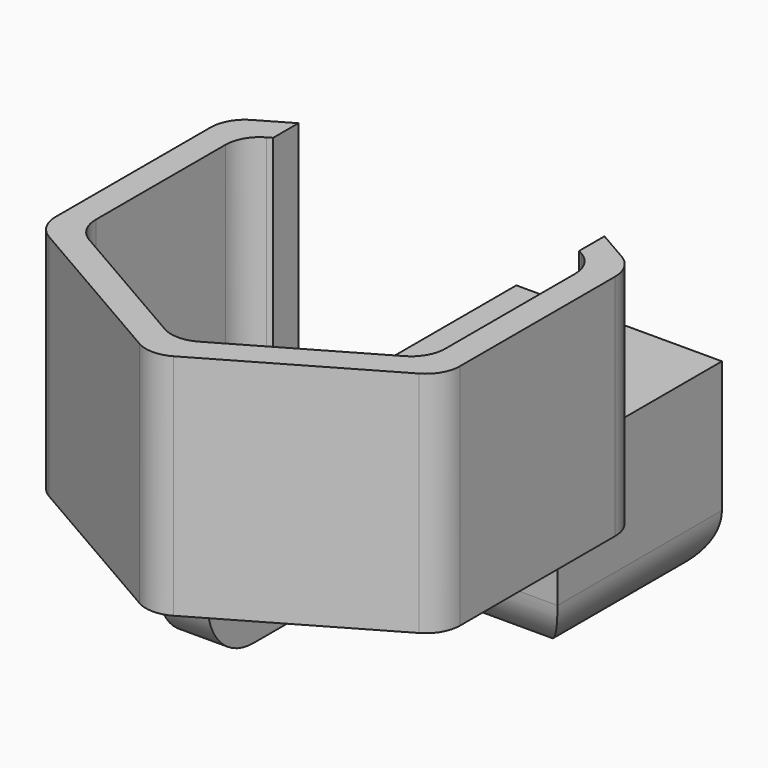
from build123d import *

# Parameters (mm, degrees)
F1_DEPTH     = 1.5
F2_DEPTH     = 20
F4_W         = 26.8
F4_H         = 20.4379309565
F5_DEPTH     = 26
F6_R         = 3
F7_R         = 0.5
F9_DEPTH     = 1.5
F10_W        = 18
F10_H        = 18
F11_DEPTH    = 15
F12_R        = 5
F13_W        = 4.3204394169
F13_H        = 29.8547168866
F14_DEPTH    = 5
F15_R        = 4.99999
F16_W        = 4.3204394169
F16_H        = 4.5489102274
F17_DEPTH    = 5
F18_T1_DEPTH = 29.218490554


# Not quite as in the source:
# - a fillet or chamfer that OpenCascade refuses, or shapes differently, is made with other operations: its cross-section is extruded or revolved along the edge and cut away or added
# - a fillet or chamfer is up to 0.001 mm smaller than in the source, because OpenCascade refuses the exact size


with BuildPart() as f1:
    # F0 (on Top) → F1 (new body)
    with BuildSketch(Plane.XY):
        Polygon((0, -17.6669182372), (15.3, -8.8334591186), (15.3, 8.8334591186), (0, 17.6669182372), (-15.3, 8.8334591186), (-15.3, -8.8334591186), align=None)
        with BuildLine():
            ThreePointArc((-6.0811183182, -8.4852813742), (-8.4852813742, -8.4852813742), (-8.4852813742, -6.0811183182))
            Line((-8.4852813742, -6.0811183182), (-6.6468037432, -4.2426406871))
            ThreePointArc((-6.6468037432, -4.2426406871), (-4.2426406871, -4.2426406871), (-4.2426406871, -6.6468037432))
            Line((-4.2426406871, -6.6468037432), (-6.0811183182, -8.4852813742))
        make_face(mode=Mode.SUBTRACT)
        with BuildLine():
            ThreePointArc((8.4852813742, -6.0811183182), (8.4852813742, -8.4852813742), (6.0811183182, -8.4852813742))
            Line((6.0811183182, -8.4852813742), (4.2426406871, -6.6468037432))
            ThreePointArc((4.2426406871, -6.6468037432), (4.2426406871, -4.2426406871), (6.6468037432, -4.2426406871))
            Line((6.6468037432, -4.2426406871), (8.4852813742, -6.0811183182))
        make_face(mode=Mode.SUBTRACT)
        with BuildLine():
            ThreePointArc((-8.4852813742, 6.0811183182), (-8.4852813742, 8.4852813742), (-6.0811183182, 8.4852813742))
            Line((-6.0811183182, 8.4852813742), (-4.2426406871, 6.6468037432))
            ThreePointArc((-4.2426406871, 6.6468037432), (-4.2426406871, 4.2426406871), (-6.6468037432, 4.2426406871))
            Line((-6.6468037432, 4.2426406871), (-8.4852813742, 6.0811183182))
        make_face(mode=Mode.SUBTRACT)
        with BuildLine():
            Line((4.2426406871, 6.6468037432), (6.0811183182, 8.4852813742))
            ThreePointArc((6.0811183182, 8.4852813742), (8.4852813742, 8.4852813742), (8.4852813742, 6.0811183182))
            Line((8.4852813742, 6.0811183182), (6.6468037432, 4.2426406871))
            ThreePointArc((6.6468037432, 4.2426406871), (4.2426406871, 4.2426406871), (4.2426406871, 6.6468037432))
        make_face(mode=Mode.SUBTRACT)
    extrude(amount=F1_DEPTH)

    # F0 (on Top) → F2 (join)
    with BuildSketch(Plane.XY):
        Polygon((-17.7, 10.2190997647), (-17.7, -10.2190997647), (0, -20.4381995293), (17.7, -10.2190997647), (17.7, 10.2190997647), (0, 20.4381995293), align=None)
        Polygon((15.3, 8.8334591186), (15.3, -8.8334591186), (0, -17.6669182372), (-15.3, -8.8334591186), (-15.3, 8.8334591186), (0, 17.6669182372), align=None, mode=Mode.SUBTRACT)
    extrude(amount=F2_DEPTH)

    # F4 (on offset) → F5 (cut)
    with BuildSketch(Plane.XZ.offset(-25)):
        with Locations((0, 11.7189654782)):
            Rectangle(F4_W, F4_H)
    extrude(amount=F5_DEPTH, mode=Mode.SUBTRACT)

    # F6
    f6_edges = [f1.edges().sort_by_distance(p)[0] for p in [
        (17.7, 10.2191, 10),
        (-17.7, 10.2191, 10),
        (-17.7, -10.2191, 10),
        (0, -20.4382, 10),
        (17.7, -10.2191, 10),
        (15.3, 8.833459, 10.75),
        (15.3, -8.833459, 10.75),
        (0, -17.666918, 10.75),
        (-15.3, -8.833459, 10.75),
        (-15.3, 8.833459, 10.75),
    ]]
    fillet(f6_edges, radius=F6_R)

    # F7
    f7_edges = [f1.edges().sort_by_distance(p)[0] for p in [
        (-13.6, 9.814955, 1.5),
        (0, 20.4382, 0.75),
        (-7.65, -13.250189, 1.5),
        (-14.898076, -8.601408, 1.5),
        (0, -17.202817, 1.5),
        (-15.3, 0, 1.5),
        (7.65, -13.250189, 1.5),
        (-14.898076, 8.601408, 1.5),
        (14.898076, -8.601408, 1.5),
        (15.3, 0, 1.5),
        (14.898076, 8.601408, 1.5),
        (13.6, 9.814955, 1.5),
    ]]
    fillet(f7_edges, radius=F7_R)

    # F8 (on face) → F9 (join)
    with BuildSketch(Plane.XY.offset(1.5)):
        with BuildLine():
            Line((-8.9667634256, 31.0121076152), (-8.9667634256, 15.2612362518))
            Line((-8.9667634256, 15.2612362518), (-0.25, 20.293861962))
            ThreePointArc((-0.25, 20.293861962), (0, 20.3608492601), (0.25, 20.293861962))
            Line((0.25, 20.293861962), (9.0332365744, 15.2228579614))
            Line((9.0332365744, 15.2228579614), (9.0332365744, 31.0121076152))
            Line((9.0332365744, 31.0121076152), (-8.9667634256, 31.0121076152))
        make_face()
    extrude(amount=-F9_DEPTH)

    # F10 (on face) → F11 (join)
    with BuildSketch(Plane(origin=(0, 0, 0), x_dir=(1, 0, 0), z_dir=(0, 0, -1))):
        with Locations((0.0332365744, -22.0121076152)):
            Rectangle(F10_W, F10_H)
    extrude(amount=F11_DEPTH)

    # F12
    f12_edges = [f1.edges().sort_by_distance(p)[0] for p in [
        (9.033237, 22.012108, -15),
        (0.033237, 13.012108, -15),
        (-8.966763, 22.012108, -15),
        (0.033237, 31.012108, -15),
    ]]
    fillet(f12_edges, radius=F12_R)

    # F13 (on face) → F14 (join)
    with BuildSketch(Plane(origin=(0, 0, 0), x_dir=(1, 0, 0), z_dir=(0, 0, -1))):
        with Locations((0.1270717476, 1.9152508281)):
            Rectangle(F13_W, F13_H)
    extrude(amount=F14_DEPTH)

    # F15 (radius 5 in the source; OpenCascade refuses exactly that, so slightly less here)
    f15_edges = [f1.edges().sort_by_distance(p)[0] for p in [
        (0.127072, -16.842609, -5),
    ]]
    fillet(f15_edges, radius=F15_R)

    # F16 (on face) → F17 (join)
    with BuildSketch(Plane(origin=(0, 0, -5), x_dir=(1, 0, 0), z_dir=(0, 0, -1))):
        with Locations((0.1270717476, -10.7376525015)):
            Rectangle(F16_W, F16_H)
    extrude(amount=F17_DEPTH)

    # F18: fillet of radius 5 on 1 edges, made by hand

    # F18_s2 → F18_t1 (cut)
    with BuildSketch(Plane.YZ.offset(-14.4821735295)):
        with BuildLine():
            ThreePointArc((8.4631973878, -5.0203897726), (9.7716225976, -8.3926702426), (13.0121076152, -10))
            Line((13.0121076152, -10), (13.0030858197, -10.0995922045))
            ThreePointArc((13.0030858197, -10.0995922045), (10.7376525015, -10.1), (8.4631973878, -10.1))
            Line((8.4631973878, -10.1), (8.3631973878, -10))
            Line((8.3631973878, -10), (8.3631973878, -5.0203897726))
            Line((8.3631973878, -5.0203897726), (8.4631973878, -5.0203897726))
        make_face()
    extrude(amount=F18_T1_DEPTH, mode=Mode.SUBTRACT)


solid = f1.part
